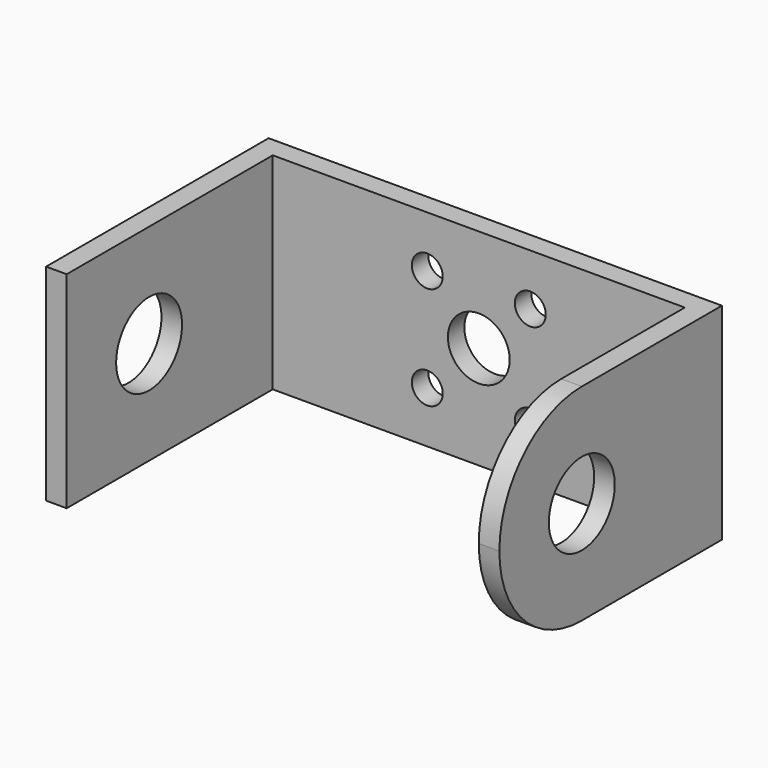
from build123d import *

# Parameters (mm, degrees)
F0_W     = 2
F0_H     = 25
F1_DEPTH = 10
F2_R     = 9.99999
F4_D     = 6
F6_D     = 3
F8_D     = 8


# Not quite as in the source:
# - a fillet or chamfer is up to 0.001 mm smaller than in the source, because OpenCascade refuses the exact size


with BuildPart() as f1:
    # F0 (on Top) → F1 (new body, symmetric)
    with BuildSketch(Plane.XY):
        with Locations((-21, -1)):
            Rectangle(F0_W, F0_H)
        Polygon((-22, 13.5), (-22, 11.5), (-20, 11.5), (20, 11.5), (22, 11.5), (22, 13.5), align=None)
        with Locations((21, -1)):
            Rectangle(F0_W, F0_H)
    extrude(amount=F1_DEPTH, both=True)

    # F2 (radius 10 in the source; OpenCascade refuses exactly that, so slightly less here)
    f2_edges = [f1.edges().sort_by_distance(p)[0] for p in [
        (21, -13.5, 10),
        (21, -13.5, -10),
    ]]
    fillet(f2_edges, radius=F2_R)

    # F4 (through all)
    with Locations(Plane(origin=(0, 13.5, 0), x_dir=(-1, 0, 0), z_dir=(0, 1, 0))):
        with Locations((0, 0)):
            Hole(F4_D / 2)

    # F6 (through all)
    with Locations(Plane(origin=(0, 13.5, 0), x_dir=(-1, 0, 0), z_dir=(0, 1, 0))):
        with Locations((-5, 5), (5, 5), (5, -5), (-5, -5)):
            Hole(F6_D / 2)

    # F8 (through all)
    with Locations(Plane.YZ.offset(22)):
        with Locations((-3.5, 0)):
            Hole(F8_D / 2)


solid = f1.part
